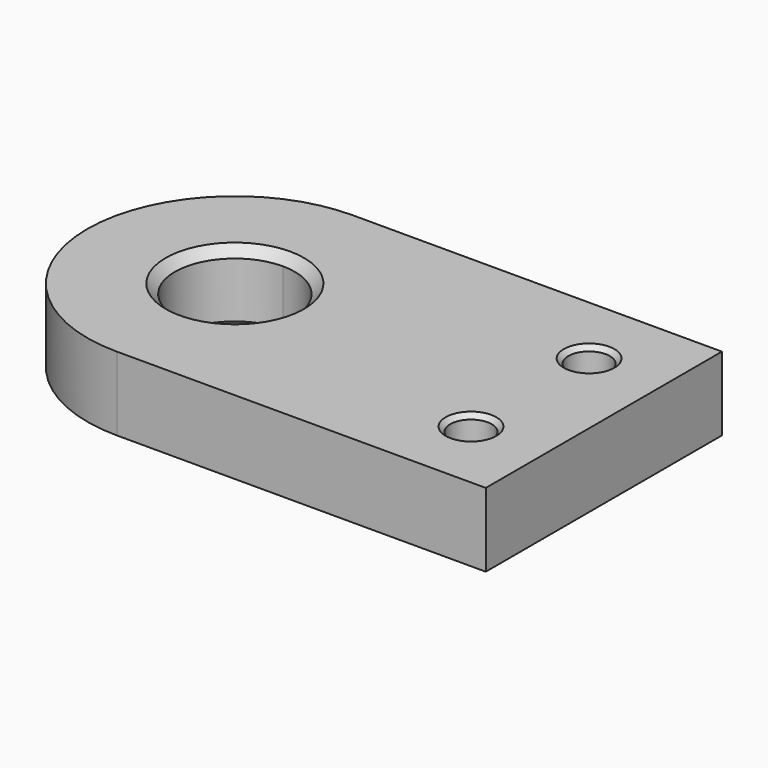
from build123d import *

# Parameters (mm, degrees)
F0_R     = 3.5687
F1_DEPTH = 12.7
F3_SIZE  = 0.79375


# Not quite as in the source:
# - a fillet or chamfer that OpenCascade refuses, or shapes differently, is made with other operations: its cross-section is extruded or revolved along the edge and cut away or added


with BuildPart() as f1:
    # F0 (on Top) → F1 (new body)
    with BuildSketch(Plane.XY):
        with BuildLine():
            Line((0, 10.31875), (0, 25.4))
            ThreePointArc((0, 25.4), (-25.4, 0), (0, -25.4))
            Line((0, -25.4), (0, -10.31875))
            ThreePointArc((0, -10.31875), (-10.31875, 0), (0, 10.31875))
        make_face()
        with BuildLine():
            ThreePointArc((0, 25.4), (17.9605122421, 17.9605122421), (25.4, 0))
            ThreePointArc((25.4, 0), (17.9605122421, -17.9605122421), (0, -25.4))
            Line((0, -25.4), (63.5, -25.4))
            Line((63.5, -25.4), (63.5, 25.4))
            Line((63.5, 25.4), (0, 25.4))
        make_face()
        with Locations((50.8, -12.7)):
            Circle(F0_R, mode=Mode.SUBTRACT)
        with Locations((50.8, 12.7)):
            Circle(F0_R, mode=Mode.SUBTRACT)
        with BuildLine():
            ThreePointArc((0, -25.4), (17.9605122421, -17.9605122421), (25.4, 0))
            ThreePointArc((25.4, 0), (17.9605122421, 17.9605122421), (0, 25.4))
            Line((0, 25.4), (0, 10.31875))
            ThreePointArc((0, 10.31875), (7.2964580984, 7.2964580984), (10.31875, 0))
            ThreePointArc((10.31875, 0), (7.2964580984, -7.2964580984), (0, -10.31875))
            Line((0, -10.31875), (0, -25.4))
        make_face()
    extrude(amount=F1_DEPTH)

    # F2: chamfer of 1.5875 on 2 edges, made by hand

    # F2_s1 → F2_t2 (revolve, cut)
    with BuildSketch(Plane.YZ):
        Polygon((10.31875, 1.5875), (11.90625, 0), (10.31875, 0), align=None)
    revolve(axis=Axis((0, 0, 0), (0, 0, -1)), mode=Mode.SUBTRACT)

    # F2_s3 → F2_t4 (revolve, cut)
    with BuildSketch(Plane.YZ):
        Polygon((10.31875, 11.1125), (11.90625, 12.7), (10.31875, 12.7), align=None)
    revolve(axis=Axis((0, 0, 12.7), (0, 0, -1)), mode=Mode.SUBTRACT)

    # F3
    f3_edges = [f1.edges().sort_by_distance(p)[0] for p in [
        (47.2313, -12.7, 0),
        (47.2313, 12.7, 0),
        (47.2313, -12.7, 12.7),
        (47.2313, 12.7, 12.7),
    ]]
    chamfer(f3_edges, length=F3_SIZE)


solid = f1.part
